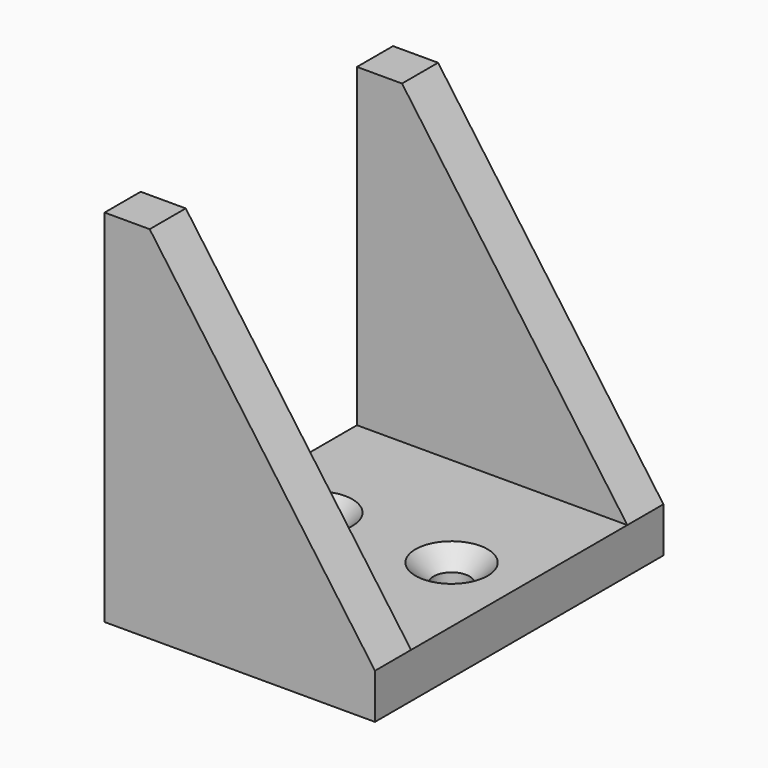
from build123d import *

# Parameters (mm, degrees)
F0_R     = 2
F1_DEPTH = 5
F3_DEPTH = 5
F5_DEPTH = 5
F6_SIZE  = 2


# Not quite as in the source:
# - a feature names something its author has since deleted; it is built from what else it names


with BuildPart() as f1:
    # F0 (on Top) → F1 (new body)
    with BuildSketch(Plane.XY):
        Polygon((-67.5038768748, 35.6870033689), (-97.5038768748, 35.6870033689), (-97.5038768748, 30.6870033689), (-97.5038768748, 0.6870033689), (-97.5038768748, -4.3129966311), (-67.5038768748, -4.3129966311), align=None)
        with Locations((-90.0038768748, 15.6870033689)):
            Circle(F0_R, mode=Mode.SUBTRACT)
        with Locations((-75.0038768748, 15.6870033689)):
            Circle(F0_R, mode=Mode.SUBTRACT)
    extrude(amount=F1_DEPTH)

    # F2 (on face) → F3 (join)
    with BuildSketch(Plane.XZ.offset(4.3129966311)):
        Polygon((-97.5038768748, 5), (-67.5038768748, 5), (-92.5038768748, 40), (-97.5038768748, 40), align=None)
    extrude(amount=-F3_DEPTH)

    # F4 (on face) → F5 (join)
    with BuildSketch(Plane(origin=(0, 35.6870033689, 0), x_dir=(-1, 0, 0), z_dir=(0, 1, 0))):
        Polygon((92.5038768748, 40), (67.5038768748, 5), (97.5038768748, 5), (97.5038768748, 40), align=None)
    extrude(amount=-F5_DEPTH)

    # F6
    f6_edges = [f1.edges().sort_by_distance(p)[0] for p in [
        (-77.003877, 15.687003, 5),
        (-92.003877, 15.687003, 5),
    ]]
    chamfer(f6_edges, length=F6_SIZE)


solid = f1.part
